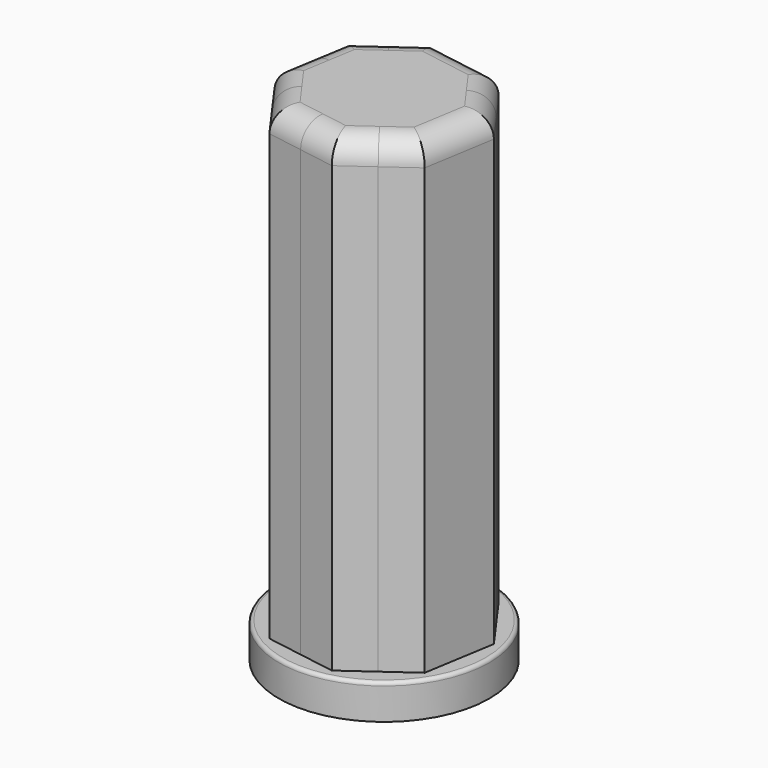
from build123d import *

# Parameters (mm, degrees)
F0_R     = 45
F1_DEPTH = 15
F3_DEPTH = 200
F5_R     = 1.5
F7_DEPTH = 10
F9_DEPTH = 2
F10_R    = 10


with BuildPart() as f1:
    # F0 (on Top) → F1 (new body)
    with BuildSketch(Plane.XY):
        Circle(F0_R)
    extrude(amount=F1_DEPTH)

    # F2 (on face) → F3 (join)
    with BuildSketch(Plane.XY.offset(15)):
        with BuildLine():
            ThreePointArc((-37.0031531736, 6.0841314261), (-31.8581593507, 19.7814984969), (-21.8630493056, 30.4673115824))
            Line((-21.8630493056, 30.4673115824), (-34.4830231078, 21.4113398267))
            Line((-34.4830231078, 21.4113398267), (-37.0031531736, 6.0841314261))
        make_face()
        with BuildLine():
            ThreePointArc((-21.8630493056, 30.4673115824), (-8.5394884365, 36.5147523235), (6.08413213, 37.0031530579))
            Line((6.08413213, 37.0031530579), (-9.2430758896, 39.5232830611))
            Line((-9.2430758896, 39.5232830611), (-21.8630493056, 30.4673115824))
        make_face()
        with BuildLine():
            ThreePointArc((6.08413213, 37.0031530579), (19.7814989367, 31.8581590776), (30.4673117702, 21.863049044))
            Line((30.4673117702, 21.863049044), (21.4113398267, 34.4830231078))
            Line((21.4113398267, 34.4830231078), (6.08413213, 37.0031530579))
        make_face()
        with BuildLine():
            ThreePointArc((30.4673117702, 21.863049044), (35.6985587341, 11.483157419), (37.5, 0))
            ThreePointArc((37.5, 0), (37.3755819089, -3.0521921581), (37.0031532283, -6.0841310937))
            Line((37.0031532283, -6.0841310937), (39.5232830611, 9.2430758896))
            Line((39.5232830611, 9.2430758896), (30.4673117702, 21.863049044))
        make_face()
        with BuildLine():
            ThreePointArc((-30.4673118862, -21.8630488823), (-36.5147523015, -8.5394885302), (-37.0031531736, 6.0841314261))
            Line((-37.0031531736, 6.0841314261), (-39.5232830611, -9.2430758896))
            Line((-39.5232830611, -9.2430758896), (-30.4673118862, -21.8630488823))
        make_face()
        with BuildLine():
            Line((-21.4113398267, -34.4830231078), (-6.084131695, -37.0031531294))
            ThreePointArc((-6.084131695, -37.0031531294), (-19.781498834, -31.8581591414), (-30.4673118862, -21.8630488823))
            Line((-30.4673118862, -21.8630488823), (-21.4113398267, -34.4830231078))
        make_face()
        with BuildLine():
            Line((9.2430758896, -39.5232830611), (21.8630489822, -30.4673118145))
            ThreePointArc((21.8630489822, -30.4673118145), (8.5394884574, -36.5147523186), (-6.084131695, -37.0031531294))
            Line((-6.084131695, -37.0031531294), (9.2430758896, -39.5232830611))
        make_face()
        with BuildLine():
            Line((34.4830231078, -21.4113398267), (37.0031532283, -6.0841310937))
            ThreePointArc((37.0031532283, -6.0841310937), (31.8581593346, -19.7814985229), (21.8630489822, -30.4673118145))
            Line((21.8630489822, -30.4673118145), (34.4830231078, -21.4113398267))
        make_face()
        with BuildLine():
            ThreePointArc((37.0031532283, -6.0841310937), (37.3755819089, -3.0521921581), (37.5, 0))
            ThreePointArc((37.5, 0), (35.6985587341, 11.483157419), (30.4673117702, 21.863049044))
            ThreePointArc((30.4673117702, 21.863049044), (19.7814989367, 31.8581590776), (6.08413213, 37.0031530579))
            ThreePointArc((6.08413213, 37.0031530579), (-8.5394884365, 36.5147523235), (-21.8630493056, 30.4673115824))
            ThreePointArc((-21.8630493056, 30.4673115824), (-31.8581593507, 19.7814984969), (-37.0031531736, 6.0841314261))
            ThreePointArc((-37.0031531736, 6.0841314261), (-36.5147523015, -8.5394885302), (-30.4673118862, -21.8630488823))
            ThreePointArc((-30.4673118862, -21.8630488823), (-19.781498834, -31.8581591414), (-6.084131695, -37.0031531294))
            ThreePointArc((-6.084131695, -37.0031531294), (8.5394884574, -36.5147523186), (21.8630489822, -30.4673118145))
            ThreePointArc((21.8630489822, -30.4673118145), (31.8581593346, -19.7814985229), (37.0031532283, -6.0841310937))
        make_face()
    extrude(amount=F3_DEPTH)

    # F5
    f5_edges = [f1.edges().sort_by_distance(p)[0] for p in [
        (-45, 0, 15),
    ]]
    fillet(f5_edges, radius=F5_R)

    # F10
    f10_edges = [f1.edges().sort_by_distance(p)[0] for p in [
        (-37.003153, 6.084132, 215),
        (-30.467311, -21.863049, 215),
        (-6.084132, -37.003153, 215),
        (21.863049, -30.467311, 215),
        (37.003153, -6.084132, 215),
        (30.467311, 21.863049, 215),
        (6.084132, 37.003153, 215),
        (-21.863049, 30.467311, 215),
    ]]
    fillet(f10_edges, radius=F10_R)


with BuildPart() as f7:
    # F6 (on face) → F7 (new body)
    with BuildSketch(Plane(origin=(0, 0, 0), x_dir=(1, 0, 0), z_dir=(0, 0, -1))):
        with BuildLine():
            ThreePointArc((-44.821869662, -4), (-45, 0), (-44.821869662, 4))
            Line((-44.821869662, 4), (-47.2203977406, 4))
            Line((-47.2203977406, 4), (-47.2203977406, -4))
            Line((-47.2203977406, -4), (-44.821869662, -4))
        make_face()
    extrude(amount=-F7_DEPTH)

    # F8 (on face) → F9 (join)
    with BuildSketch(Plane(origin=(-47.2203977406, 0, 0), x_dir=(0, -1, 0), z_dir=(-1, 0, 0))):
        with BuildLine():
            Line((0, 5), (0, 6.5))
            ThreePointArc((0, 6.5), (-1.0606601718, 6.0606601718), (-1.5, 5))
            Line((-1.5, 5), (0, 5))
        make_face()
        with BuildLine():
            ThreePointArc((1.5, 5), (1.0606601718, 6.0606601718), (0, 6.5))
            Line((0, 6.5), (0, 5))
            Line((0, 5), (1.5, 5))
        make_face()
        with BuildLine():
            Line((1.5, 5), (0, 5))
            Line((0, 5), (0, 3.5))
            ThreePointArc((0, 3.5), (1.0606601718, 3.9393398282), (1.5, 5))
        make_face()
        with BuildLine():
            Line((0, 3.5), (0, 5))
            Line((0, 5), (-1.5, 5))
            ThreePointArc((-1.5, 5), (-1.0606601718, 3.9393398282), (0, 3.5))
        make_face()
    extrude(amount=F9_DEPTH)


solid = Compound([f1.part, f7.part])
